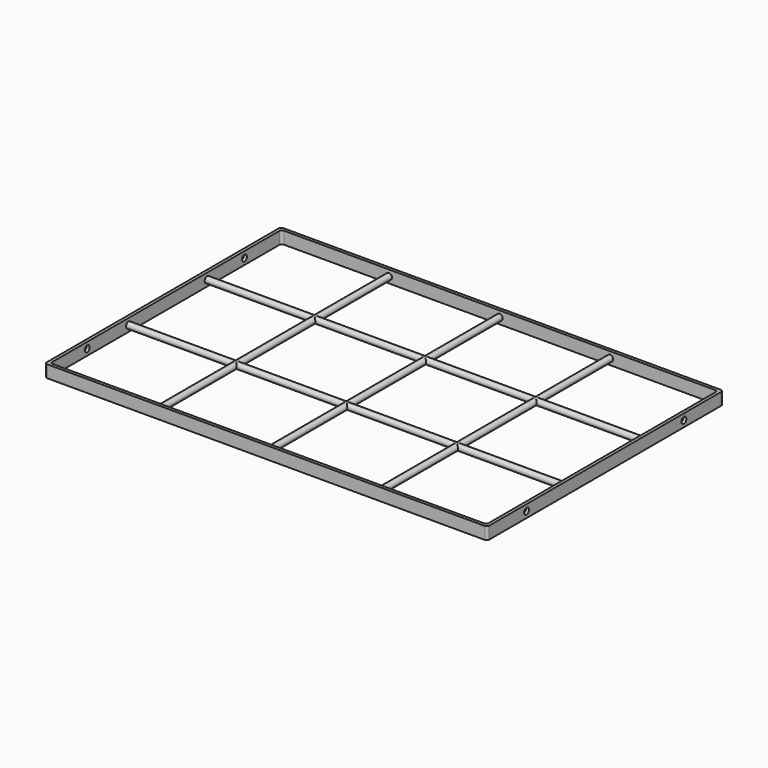
from build123d import *

# Parameters (mm, degrees)
F0_W      = 914.4
F0_H      = 609.6
F0_W_2    = 901.7
F0_H_2    = 596.9
F1_DEPTH  = 25.4
F2_R      = 5.08
F3_R      = 6.35
F4_DEPTH  = 901.7
F5_R      = 6.35
F6_DEPTH  = 596.9
F8_D      = 12.7
F8_DEPTH  = 6.35
F8_TIP    = 3.8154649308
F10_D     = 12.7
F10_DEPTH = 6.35
F10_TIP   = 3.8154649308


# Not quite as in the source:
# - a length typed as a fraction of an inch, garbled in the dataset ("3 / 203.2 mm" for 3/8 in), is restored


with BuildPart() as f1:
    # F0 (on Top) → F1 (new body)
    with BuildSketch(Plane.XY):
        with Locations((457.2, -304.8)):
            Rectangle(F0_W, F0_H)
        with Locations((457.2, -304.8)):
            Rectangle(F0_W_2, F0_H_2, mode=Mode.SUBTRACT)
    extrude(amount=F1_DEPTH)

    # F2
    f2_edges = [f1.edges().sort_by_distance(p)[0] for p in [
        (914.4, 0, 12.7),
        (908.05, -603.25, 12.7),
        (0, 0, 12.7),
        (6.35, -603.25, 12.7),
        (914.4, -609.6, 12.7),
        (0, -609.6, 12.7),
        (908.05, -6.35, 12.7),
        (6.35, -6.35, 12.7),
    ]]
    fillet(f2_edges, radius=F2_R)

    # F8
    with Locations(Plane(origin=(0, 0, 0), x_dir=(0, -1, 0), z_dir=(-1, 0, 0))):
        with Locations((101.6, 12.7), (508, 12.7)):
            Hole(F8_D / 2, depth=F8_DEPTH)
            with Locations((0, 0, -(F8_DEPTH + F8_TIP / 2))):  # 118° drill point
                Cone(0, F8_D / 2, F8_TIP, mode=Mode.SUBTRACT)

    # F10
    with Locations(Plane.YZ.offset(914.4)):
        with Locations((-508, 12.7), (-101.6, 12.7)):
            Hole(F10_D / 2, depth=F10_DEPTH)
            with Locations((0, 0, -(F10_DEPTH + F10_TIP / 2))):  # 118° drill point
                Cone(0, F10_D / 2, F10_TIP, mode=Mode.SUBTRACT)


with BuildPart() as f4:
    # F3 (on face) → F4 (new body, through all)
    with BuildSketch(Plane.YZ.offset(6.35)):
        with Locations((-401.32, 12.7)):
            Circle(F3_R)
    extrude(amount=F4_DEPTH)


with BuildPart() as f4b:
    # F3 (on face) → F4, piece 2 (new body, through all)
    with BuildSketch(Plane.YZ.offset(6.35)):
        with Locations((-198.12, 12.7)):
            Circle(F3_R)
    extrude(amount=F4_DEPTH)


with BuildPart() as f6:
    # F5 (on face) → F6 (new body, through all)
    with BuildSketch(Plane.XZ.offset(6.35)):
        with Locations((228.6, 12.7)):
            Circle(F5_R)
    extrude(amount=F6_DEPTH)


with BuildPart() as f6b:
    # F5 (on face) → F6, piece 2 (new body, through all)
    with BuildSketch(Plane.XZ.offset(6.35)):
        with Locations((457.2, 12.7)):
            Circle(F5_R)
    extrude(amount=F6_DEPTH)


with BuildPart() as f6c:
    # F5 (on face) → F6, piece 3 (new body, through all)
    with BuildSketch(Plane.XZ.offset(6.35)):
        with Locations((685.8, 12.7)):
            Circle(F5_R)
    extrude(amount=F6_DEPTH)


solid = Compound([f1.part, f4.part, f4b.part, f6.part, f6b.part, f6c.part])
